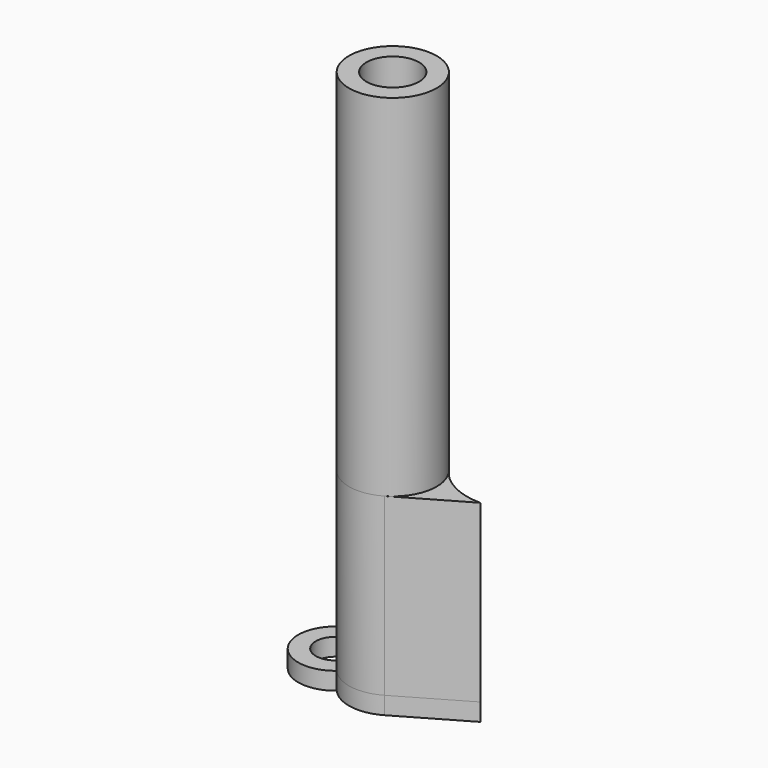
from build123d import *
from build123d import SkipClean  # not in build123d's __all__

# Parameters (mm, degrees)
F1_DEPTH = 20
F2_R     = 5
F2_R_2   = 3
F3_DEPTH = 40
F4_R     = 3
F5_DEPTH = 2
F7_DEPTH = 2


with BuildPart() as f1:
    # F0 (on Top) → F1 (new body)
    with BuildSketch(Plane.XY):
        with BuildLine():
            ThreePointArc((3.6918747639, 3.3719520649), (-1.8084006996, 4.661511226), (-5, 0))
            ThreePointArc((-5, 0), (-2.4980082156, -4.3312763656), (2.503981982, -4.327825578))
            Line((2.503981982, -4.327825578), (9.9840974016, 0))
            ThreePointArc((9.9840974016, 0), (6.8273158844, 0.6909487043), (4.2478112604, 2.637441847))
            ThreePointArc((4.2478112604, 2.637441847), (3.9586403918, 2.9962179106), (3.6918747639, 3.3719520649))
        make_face()
        with BuildLine():
            ThreePointArc((-3, 0), (0, 3), (3, 0))
            ThreePointArc((3, 0), (0, -3), (-3, 0))
        make_face(mode=Mode.SUBTRACT)
    extrude(amount=F1_DEPTH)

    # F2 (on face) → F3 (join)
    with BuildSketch(Plane.XY.offset(20)):
        Circle(F2_R)
        Circle(F2_R_2, mode=Mode.SUBTRACT)
    extrude(amount=F3_DEPTH)

    # F4 (on face) → F5 (join)
    with BuildSketch(Plane(origin=(0, 0, 0), x_dir=(1, 0, 0), z_dir=(0, 0, -1))):
        with BuildLine():
            ThreePointArc((3.6918747639, -3.3719520649), (6.414709273, -0.8961214102), (9.9840974016, 0))
            Line((9.9840974016, 0), (2.503981982, 4.327825578))
            ThreePointArc((2.503981982, 4.327825578), (-5, 0), (2.503981982, -4.327825578))
            ThreePointArc((2.503981982, -4.327825578), (3.1345787192, -3.8954353098), (3.6918747639, -3.3719520649))
        make_face()
        Circle(F4_R, mode=Mode.SUBTRACT)
        with BuildLine():
            Line((2.503981982, -4.327825578), (9.9840974016, 0))
            ThreePointArc((9.9840974016, 0), (6.414709273, -0.8961214102), (3.6918747639, -3.3719520649))
            ThreePointArc((3.6918747639, -3.3719520649), (3.1345787192, -3.8954353098), (2.503981982, -4.327825578))
        make_face()
    with SkipClean():  # cleaning this boolean's faces spoils the solid; the shape is the same uncleaned
        extrude(amount=F5_DEPTH)

    # F6 (on face) → F7 (join)
    with BuildSketch(Plane(origin=(0, 0, -2), x_dir=(1, 0, 0), z_dir=(0, 0, -1))):
        with BuildLine():
            ThreePointArc((-4.7696960071, -1.5), (-8.7790290978, 0), (-4.7696960071, 1.5))
            ThreePointArc((-4.7696960071, 1.5), (-4.3575549598, 2.4518798446), (-3.7578759927, 3.2982371084))
            ThreePointArc((-3.7578759927, 3.2982371084), (-10.7790290978, 0), (-3.7578759927, -3.2982371084))
            ThreePointArc((-3.7578759927, -3.2982371084), (-4.3575549598, -2.4518798446), (-4.7696960071, -1.5))
        make_face()
    with SkipClean():  # cleaning this boolean's faces spoils the solid; the shape is the same uncleaned
        extrude(amount=-F7_DEPTH)


solid = f1.part
